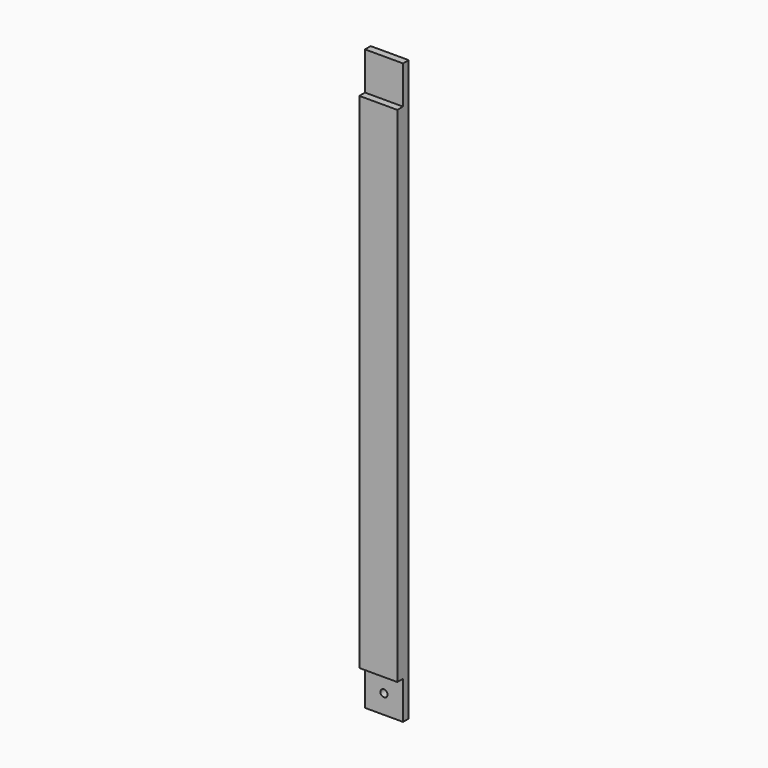
from build123d import *

# Parameters (mm, degrees)
F0_W     = 50.8
F0_H     = 19.05
F1_DEPTH = 774.7
F2_W     = 122.43557321
F2_H     = 50.8
F2_W_2   = 343.1604206562
F3_DEPTH = 25.4
F4_R     = 4.7625
F5_DEPTH = 25.4


# Not quite as in the source:
# - a feature names something its author has since deleted; it is built from what else it names


with BuildPart() as f1:
    # F0 (on Top) → F1 (new body)
    with BuildSketch(Plane.XY):
        Rectangle(F0_W, F0_H)
    extrude(amount=F1_DEPTH)

    # F2 (on Front) → F3 (cut)
    with BuildSketch(Plane.XZ):
        with Locations((22.4465244144, 25.4)):
            Rectangle(F2_W, F2_H)
        with Locations((-38.7818217278, 749.3)):
            Rectangle(F2_W_2, F2_H)
    extrude(amount=F3_DEPTH, mode=Mode.SUBTRACT)

    # F4 (on Front) → F5 (cut)
    with BuildSketch(Plane.XZ):
        with Locations((0, 25.4)):
            Circle(F4_R)
    extrude(amount=-F5_DEPTH, mode=Mode.SUBTRACT)


solid = f1.part
